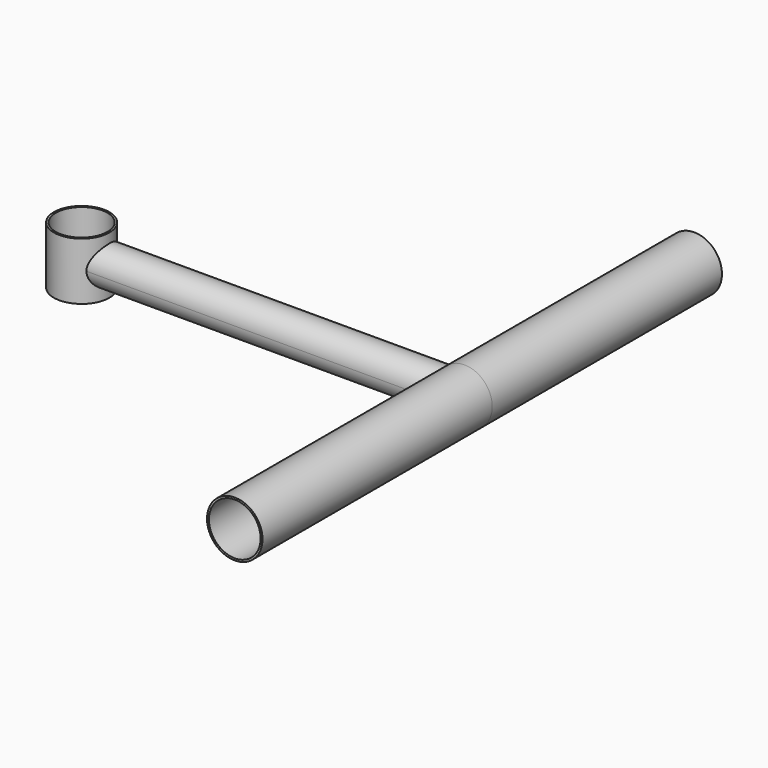
from build123d import *

# Parameters (mm, degrees)
F0_R          = 14.5
F0_R_2        = 13.5
F1_DEPTH      = 30
F3_DEPTH      = 200
F4_END_RADIUS = 13.5
F3_FACE_R     = 10
F3_FACE_R_2   = 9
F4_REACH      = 228.2852713475
F6_DEPTH      = 150
F8_END_RADIUS = 13.5
F3_FACE1_R    = 10
F3_FACE1_R_2  = 9
F8_REACH      = 242.7852713475


with BuildPart() as f1:
    # F0 (on Top) → F1 (new body)
    with BuildSketch(Plane.XY):
        Circle(F0_R)
        Circle(F0_R_2, mode=Mode.SUBTRACT)
    extrude(amount=F1_DEPTH)

    # F2 (on Right) → F3 (join)
    with BuildSketch(Plane.YZ):
        with BuildLine():
            ThreePointArc((10, 15), (-7.0710678119, 22.0710678119), (0, 5))
            ThreePointArc((0, 5), (7.0710678119, 7.9289321881), (10, 15))
        make_face()
        with BuildLine():
            ThreePointArc((9, 15), (6.3639610307, 8.6360389693), (0, 6))
            ThreePointArc((0, 6), (-6.3639610307, 21.3639610307), (9, 15))
        make_face(mode=Mode.SUBTRACT)
    extrude(amount=F3_DEPTH)

    f4_end = (Plane(origin=(0, 0, 15), x_dir=(-1, 0, 0), z_dir=(0, 0, -1)) * Cylinder(F4_END_RADIUS, 893.6117311859, mode=Mode.PRIVATE)).faces().sort_by_distance((-13.5, 0, 15))[0]
    # F3_face (on face) → F4 (cut, up to the whole of a round face its end follows)
    with BuildSketch(Plane(origin=(0, 0, 15), x_dir=(0, 1, 0), z_dir=(-1, 0, 0))):
        Circle(F3_FACE_R)
        Circle(F3_FACE_R_2, mode=Mode.SUBTRACT)
    f4_long = extrude(amount=-F4_REACH, mode=Mode.PRIVATE)
    add(split(f4_long, bisect_by=f4_end, keep=Keep.BOTTOM, mode=Mode.PRIVATE), mode=Mode.SUBTRACT)

    # F5 (on Front) → F6 (join)
    with BuildSketch(Plane.XZ):
        with BuildLine():
            ThreePointArc((214.5, 15), (200, 29.5), (185.5, 15))
            ThreePointArc((185.5, 15), (200, 0.5), (214.5, 15))
        make_face()
        with BuildLine():
            ThreePointArc((213.5, 15), (200, 1.5), (186.5, 15))
            ThreePointArc((186.5, 15), (200, 28.5), (213.5, 15))
        make_face(mode=Mode.SUBTRACT)
    extrude(amount=F6_DEPTH)

    # F7: F1 across plane


with BuildPart() as f1_1:
    add(f1.part)
    add(f1.part.mirror(Plane.XZ))

    f8_end = (Plane(origin=(200, 0, 15), x_dir=(0, 0, 1), z_dir=(0, 1, 0)) * Cylinder(F8_END_RADIUS, 1242.7785728256, mode=Mode.PRIVATE)).faces().sort_by_distance((186.5, -146.9757976235, 15))[0]
    # F3_face1 (on face) → F8 (cut, up to the whole of a round face its end follows)
    with BuildSketch(Plane(origin=(200, 0, 15), x_dir=(0, 1, 0), z_dir=(1, 0, 0))):
        Circle(F3_FACE1_R)
        Circle(F3_FACE1_R_2, mode=Mode.SUBTRACT)
    f8_long = extrude(amount=-F8_REACH, mode=Mode.PRIVATE)
    add(split(f8_long, bisect_by=f8_end, keep=Keep.BOTTOM, mode=Mode.PRIVATE), mode=Mode.SUBTRACT)


solid = f1_1.part
